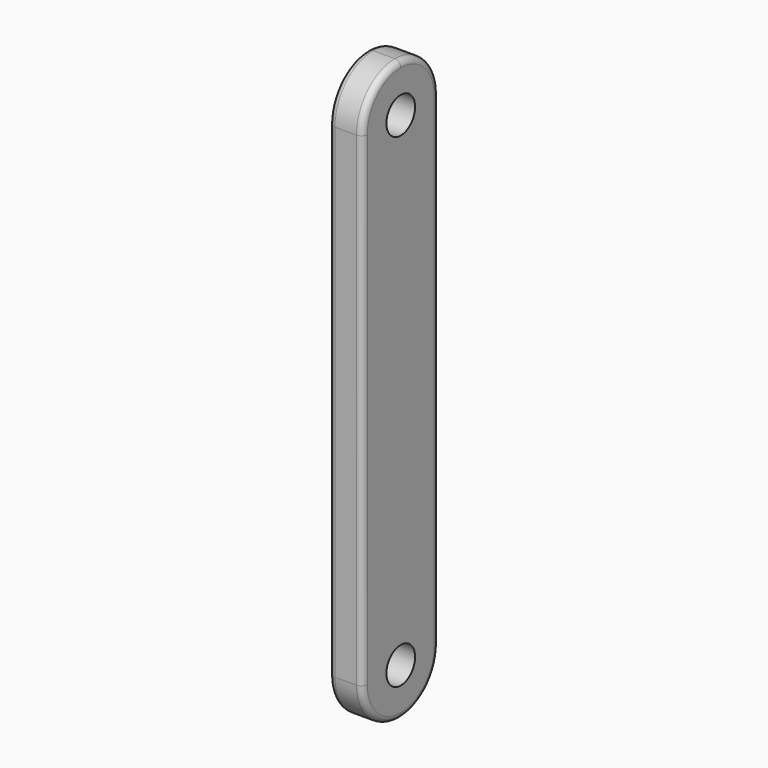
from build123d import *

# Parameters (mm, degrees)
F0_W     = 2.8
F0_H     = 8
F1_DEPTH = 48.5
F2_R     = 3.99999
F3_R     = 1.5
F4_DEPTH = 5
F5_R     = 0.5


# Not quite as in the source:
# - a fillet or chamfer is up to 0.001 mm smaller than in the source, because OpenCascade refuses the exact size


with BuildPart() as f1:
    # F0 (on Top) → F1 (new body)
    with BuildSketch(Plane.XY):
        Rectangle(F0_W, F0_H)
    extrude(amount=F1_DEPTH)

    # F2 (radius 4 in the source; OpenCascade refuses exactly that, so slightly less here)
    f2_edges = [f1.edges().sort_by_distance(p)[0] for p in [
        (0, 4, 0),
        (0, -4, 0),
        (0, -4, 48.5),
        (0, 4, 48.5),
    ]]
    fillet(f2_edges, radius=F2_R)

    # F3 (on face) → F4 (cut)
    with BuildSketch(Plane(origin=(-1.4, 0, 0), x_dir=(0, -1, 0), z_dir=(-1, 0, 0))):
        with Locations((0, 4)):
            Circle(F3_R)
        with Locations((0, 44.5)):
            Circle(F3_R)
    extrude(amount=-F4_DEPTH, mode=Mode.SUBTRACT)

    # F5
    f5_edges = [f1.edges().sort_by_distance(p)[0] for p in [
        (-1.4, 4, 24.25),
        (1.4, 4, 24.25),
    ]]
    fillet(f5_edges, radius=F5_R)


solid = f1.part
